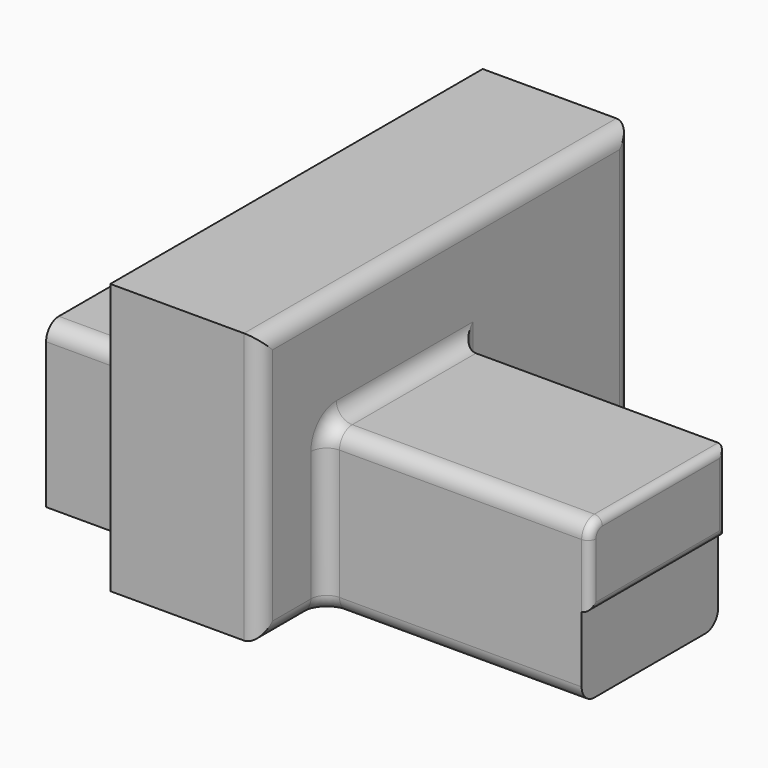
from build123d import *

# Parameters (mm, degrees)
F0_W     = 173.5329478979
F0_H     = 54.4529519975
F1_DEPTH = 25.4
F2_R     = 5.08
F3_R     = 2.54
F4_W     = 47.7339737117
F4_H     = 148.616027087
F5_DEPTH = 60.198
F6_DEPTH = 26.162
F7_R     = 5.08


with BuildPart() as f1:
    # F0 (on Top) → F1 (new body)
    with BuildSketch(Plane.XY):
        with Locations((45.8968058228, 4.7943573445)):
            Rectangle(F0_W, F0_H)
    extrude(amount=F1_DEPTH)

    # F2
    f2_edges = [f1.edges().sort_by_distance(p)[0] for p in [
        (45.896806, -22.432119, 25.4),
    ]]
    fillet(f2_edges, radius=F2_R)

    # F3
    f3_edges = [f1.edges().sort_by_distance(p)[0] for p in [
        (132.66328, -22.432119, 10.16),
        (132.66328, -20.944221, 23.912102),
        (132.66328, 4.794357, 0),
        (132.66328, 7.334357, 25.4),
        (132.66328, 32.020833, 12.7),
    ]]
    fillet(f3_edges, radius=F3_R)

    # F4 (on Top) → F5 (join)
    with BuildSketch(Plane.XY):
        with Locations((23.8669868559, 26.4220479876)):
            Rectangle(F4_W, F4_H)
    extrude(amount=F5_DEPTH)

    # F6 (add): a face of the model
    f6_faces = [f1.faces().sort_by_distance(p)[0] for p in [
        (37.8680200683, 15.9075868005, 0),
    ]]
    extrude(f6_faces, amount=F6_DEPTH)

    # F7
    f7_edges = [f1.edges().sort_by_distance(p)[0] for p in [
        (47.733974, -47.885966, 17.018),
        (47.733974, -35.159042, -26.162),
        (47.733974, -22.432119, -2.921),
        (47.733974, -20.944221, 23.912102),
        (47.733974, 7.334357, 25.4),
        (47.733974, 32.020833, -0.381),
        (47.733974, 66.375447, -26.162),
        (47.733974, 100.730062, 17.018),
        (47.733974, 26.422048, 60.198),
        (88.928627, -22.432119, -26.162),
        (88.928627, 32.020833, -26.162),
    ]]
    fillet(f7_edges, radius=F7_R)


solid = f1.part
